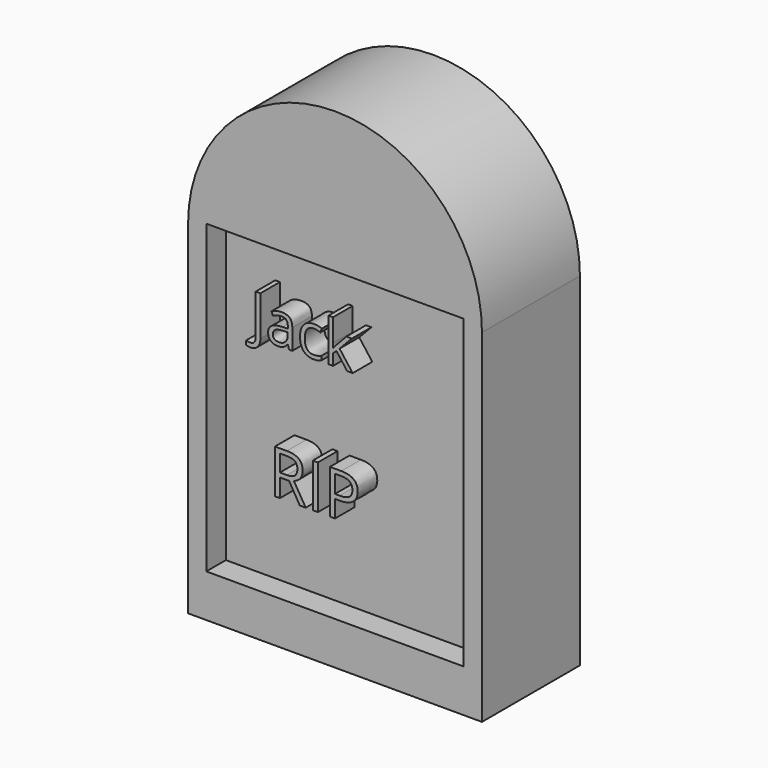
from build123d import *

# Parameters (mm, degrees)
F1_DEPTH       = 101.6
F2_W           = 266.7
F2_H           = 317.5
F3_DEPTH       = 25.4
F4_TEXT_SIZE   = 58.4634227885
F4_TEXT_SIZE_2 = 63.6219564411
F5_DEPTH       = 25.4


# Not quite as in the source:
# - Text() gives the source's letters only with a copy of the font that has no kerning and outlines rounded to 1/6400 em; it was checked with that copy


with BuildPart() as f1:
    # F0 (on Front) → F1 (new body)
    with BuildSketch(Plane.XZ):
        with BuildLine():
            Line((-180.0206861973, 282.6197302103), (-180.0206861973, -72.9802697897))
            Line((-180.0206861973, -72.9802697897), (124.7793138027, -72.9802697897))
            Line((124.7793138027, -72.9802697897), (124.7793138027, 282.6197302103))
            ThreePointArc((124.7793138027, 282.6197302103), (-27.6206861973, 435.0197302103), (-180.0206861973, 282.6197302103))
        make_face()
    extrude(amount=F1_DEPTH)

    # F2 (on face) → F3 (join)
    with BuildSketch(Plane.XZ.offset(101.6)):
        with BuildLine():
            ThreePointArc((124.7793138027, 282.6197302103), (-27.6206861973, 435.0197302103), (-180.0206861973, 282.6197302103))
            Line((-180.0206861973, 282.6197302103), (-180.0206861973, -72.9802697897))
            Line((-180.0206861973, -72.9802697897), (124.7793138027, -72.9802697897))
            Line((124.7793138027, -72.9802697897), (124.7793138027, 282.6197302103))
        make_face()
        with Locations((-27.7529622912, 130.2197302103)):
            Rectangle(F2_W, F2_H, mode=Mode.SUBTRACT)
    extrude(amount=F3_DEPTH)

    # F4 (on face) → F5 (join)
    with BuildSketch(Plane.XZ.offset(101.6)):
        with Locations((-115.3247579932, 201.8538564444)):
            Text('Jack', F4_TEXT_SIZE, font='Open Sans', text_align=(TextAlign.LEFT, TextAlign.BOTTOM))
        with Locations((-96.2282091172, 63.1923824549)):
            Text('RIP', F4_TEXT_SIZE_2, font='Open Sans', text_align=(TextAlign.LEFT, TextAlign.BOTTOM))
    extrude(amount=F5_DEPTH)


solid = f1.part
